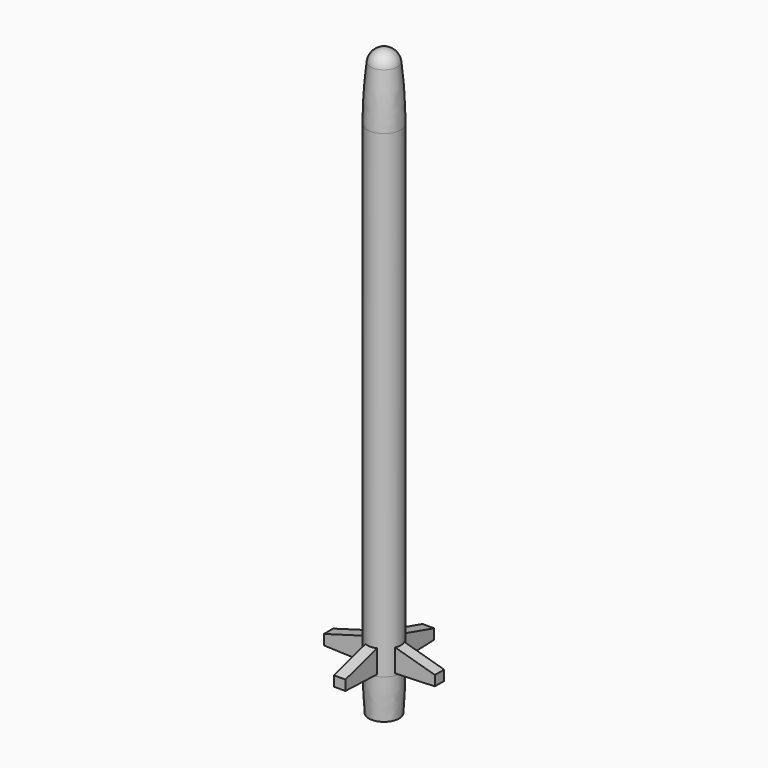
from build123d import *

# Parameters (mm, degrees)
F3_DEPTH = 0.2
F4_COUNT = 4


# Not quite as in the source:
# - a feature names something its author has since deleted; it is built from what else it names


with BuildPart() as f1:
    # F0 (on Front) → F1 (revolve)
    with BuildSketch(Plane.XZ):
        with BuildLine():
            Line((0, 20.1388888889), (0, 0))
            Line((0, 0), (0.5208333333, 0))
            ThreePointArc((0.5208333333, 0), (0.5624944489, 0.6938891109), (0.5763888889, 1.3888888889))
            Line((0.5763888889, 1.3888888889), (0.5763888889, 17.8472222222))
            ThreePointArc((0.5763888889, 17.8472222222), (0.5492348486, 18.7862912781), (0.467863469, 19.7222222222))
            ThreePointArc((0.467863469, 19.7222222222), (0.3132520298, 20.01962212), (0, 20.1388888889))
        make_face()
    revolve(axis=Axis((0, 0, 10.0694444444), (0, 0, 1)))

    # F2 (on Front) → F3 (join, symmetric)
    with BuildSketch(Plane.XZ):
        Polygon((0, 11.1135402694), (0, 1.4373737374), (1.9097222222, 1.5068181818), (1.9097222222, 1.854040404), (0.4, 2.2865129156), (0.4, 11.3888888889), align=None)
    extrude(amount=F3_DEPTH, both=True)

    # F4: F1 ×4 about axis
    f4_axis = Axis((0, 0, 1.3888888889), (0, 0, 1))


with BuildPart() as f1_1:
    add(f1.part)
    for i in range(1, F4_COUNT):
        add(f1.part.rotate(f4_axis, i * 360 / F4_COUNT))


solid = f1_1.part
